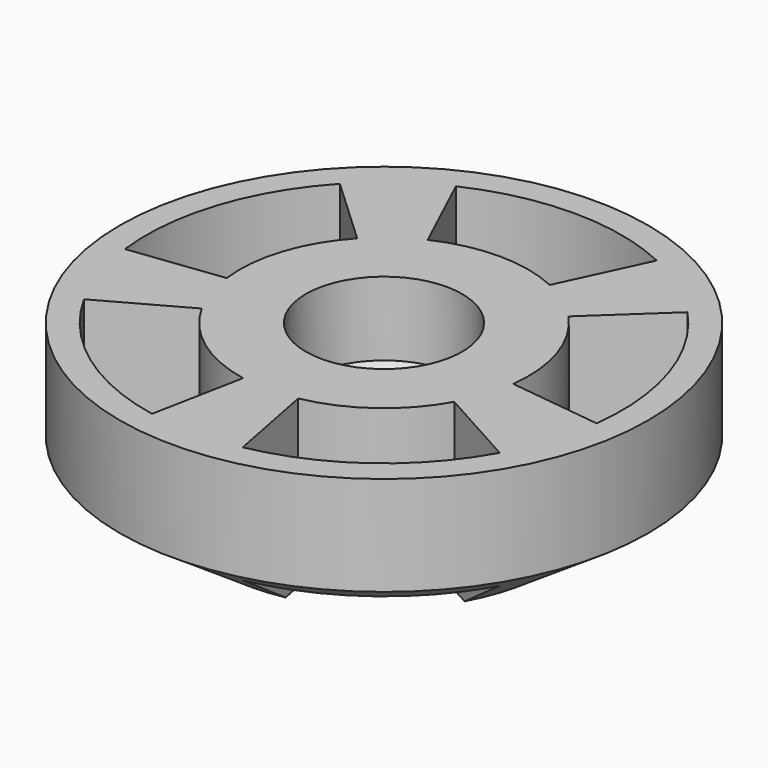
from build123d import *

# Parameters (mm, degrees)
F0_R      = 50.675
F1_DEPTH  = 95.25
F6_R      = 64.2548627896
F7_DEPTH  = 63.5
F10_DEPTH = 31.751


# Not quite as in the source:
# - a feature of the source that left no trace in its solid (it failed there, or was rolled back) is left out


with BuildPart() as f1:
    # F0 (on Top) → F1 (new body)
    with BuildSketch(Plane.XY):
        Circle(F0_R)
    extrude(amount=F1_DEPTH)

    # F2 (on Front) → F3 (revolve, cut)
    with BuildSketch(Plane.XZ):
        Polygon((-50.6984, 0), (-31.75, 0), (-50.6984, 12.7), align=None)
    revolve(axis=Axis((0, 0, 21.0587424167), (0, 0, 1)), mode=Mode.SUBTRACT)

    # F4 (on Front) → F5 (revolve, cut)
    with BuildSketch(Plane.XZ):
        Polygon((0, 0.6), (0, 108.2893535495), (-15, 108.2893535495), (-15, 17.6), (-3.5, 0.6), align=None)
    revolve(axis=Axis((0, 0, 54.4446767747), (0, 0, -1)), mode=Mode.SUBTRACT)

    # F6 (on face) → F7 (cut)
    with BuildSketch(Plane.XY.offset(95.25)):
        Circle(F6_R)
    extrude(amount=-F7_DEPTH, mode=Mode.SUBTRACT)

    # F9 (on face) → F10 (cut, through all)
    with BuildSketch(Plane.XY.offset(31.75)):
        with BuildLine():
            ThreePointArc((-11.7065258502, 25.1047257009), (0, 27.7), (11.7065258502, 25.1047257009))
            Line((11.7065258502, 25.1047257009), (19.2692796441, 41.3231035499))
            ThreePointArc((19.2692796441, 41.3231035499), (0, 45.595), (-19.2692796441, 41.3231035499))
            Line((-19.2692796441, 41.3231035499), (-11.7065258502, 25.1047257009))
        make_face()
        with BuildLine():
            ThreePointArc((-27.4935284005, -3.3757808123), (-26.3442655014, 8.5597707442), (-20.2584975349, 18.8913545737))
            Line((-20.2584975349, 18.8913545737), (-33.3460720253, 31.095715227))
            ThreePointArc((-33.3460720253, 31.095715227), (-43.3634218605, 14.0896298585), (-45.2551417841, -5.5566327126))
            Line((-45.2551417841, -5.5566327126), (-27.4935284005, -3.3757808123))
        make_face()
        with BuildLine():
            ThreePointArc((-5.2854091719, -27.1910729815), (-16.2816514885, -22.4097707442), (-24.2269658878, -13.4292264808))
            Line((-24.2269658878, -13.4292264808), (-39.878285547, -22.1048946351))
            ThreePointArc((-39.878285547, -22.1048946351), (-26.8000685783, -36.8871298585), (-8.6999361442, -44.7572914293))
            Line((-8.6999361442, -44.7572914293), (-5.2854091719, -27.1910729815))
        make_face()
        with BuildLine():
            ThreePointArc((24.2269658878, -13.4292264808), (16.2816514885, -22.4097707442), (5.2854091719, -27.1910729815))
            Line((5.2854091719, -27.1910729815), (8.6999361442, -44.7572914293))
            ThreePointArc((8.6999361442, -44.7572914293), (26.8000685783, -36.8871298585), (39.878285547, -22.1048946351))
            Line((39.878285547, -22.1048946351), (24.2269658878, -13.4292264808))
        make_face()
        with BuildLine():
            ThreePointArc((20.2584975349, 18.8913545737), (26.3442655014, 8.5597707442), (27.4935284005, -3.3757808123))
            Line((27.4935284005, -3.3757808123), (45.2551417841, -5.5566327126))
            ThreePointArc((45.2551417841, -5.5566327126), (43.3634218605, 14.0896298585), (33.3460720253, 31.095715227))
            Line((33.3460720253, 31.095715227), (20.2584975349, 18.8913545737))
        make_face()
    extrude(amount=-F10_DEPTH, mode=Mode.SUBTRACT)


solid = f1.part
